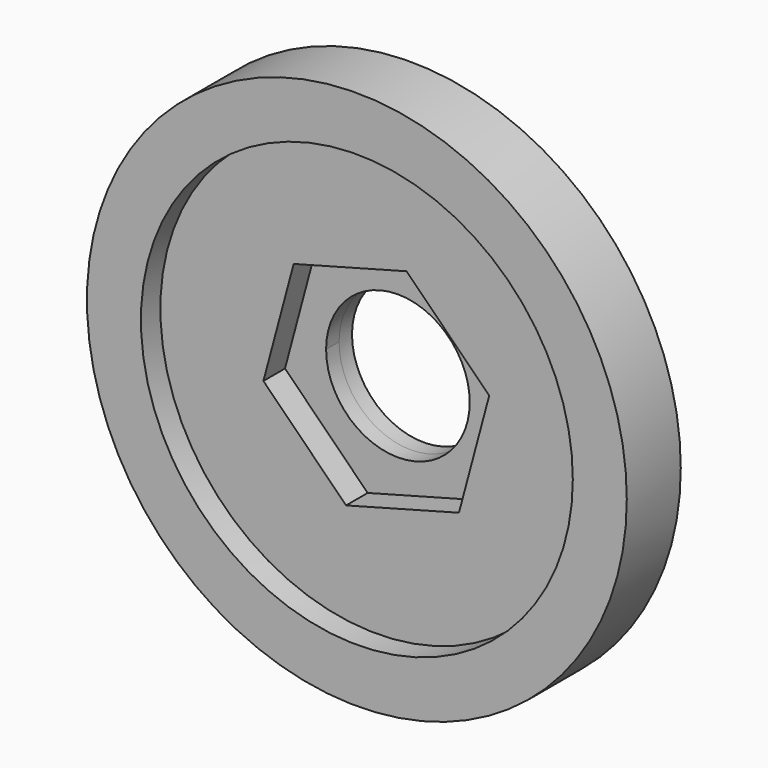
from build123d import *

# Parameters (mm, degrees)
F0_R     = 12.7
F0_R_2   = 10.16
F1_DEPTH = 3.175
F2_DEPTH = 2.032
F0_R_3   = 3.3782
F3_DEPTH = 0.762
F4_R     = 8.4455
F5_DEPTH = 0.762
F7_D     = 6.7564


# Not quite as in the source:
# - the program builds the solid bodies; features that only make, move or delete a surface that nothing else refers to are left out


with BuildPart() as f1:
    # F0 (on Front) → F1 (new body)
    with BuildSketch(Plane.XZ):
        Circle(F0_R)
        Circle(F0_R_2, mode=Mode.SUBTRACT)
    extrude(amount=F1_DEPTH)

    # F0 (on Front) → F2 (join)
    with BuildSketch(Plane.XZ):
        Circle(F0_R_2)
        Polygon((1.4233928974, 5.3116902648), (5.3117551551, 1.4231507237), (3.8883622577, -3.8885395411), (-1.4233928974, -5.3116902648), (-5.3117551551, -1.4231507237), (-3.8883622577, 3.8885395411), align=None, mode=Mode.SUBTRACT)
    extrude(amount=F2_DEPTH)

    # F0 (on Front) → F3 (join)
    with BuildSketch(Plane.XZ):
        Polygon((3.8883622577, -3.8885395411), (5.3117551551, 1.4231507237), (1.4233928974, 5.3116902648), (-3.8883622577, 3.8885395411), (-5.3117551551, -1.4231507237), (-1.4233928974, -5.3116902648), align=None)
        Circle(F0_R_3, mode=Mode.SUBTRACT)
    extrude(amount=F3_DEPTH)

    # F4 (on face) → F5 (join)
    with BuildSketch(Plane.XZ):
        Circle(F4_R)
    extrude(amount=-F5_DEPTH)

    # F7 (through all)
    with Locations(Plane.XZ):
        with Locations((0, 0)):
            Hole(F7_D / 2)


solid = f1.part
